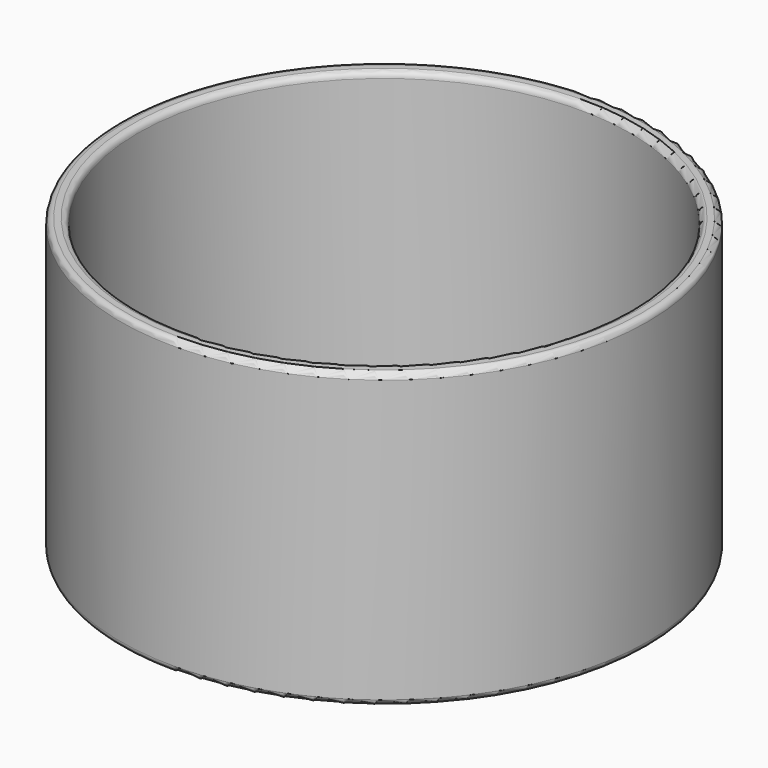
from build123d import *

# Parameters (mm, degrees)
F0_R     = 57.15
F1_DEPTH = 5.08
F2_R     = 1.27
F5_E1_W  = 63.5
F5_E1_H  = 3.81
F7_R     = 1.26999
F8_R     = 1.27


# Not quite as in the source:
# - a fillet or chamfer is up to 0.001 mm smaller than in the source, because OpenCascade refuses the exact size


with BuildPart() as f1:
    # F0 (on Top) → F1 (new body)
    with BuildSketch(Plane.XY):
        Circle(F0_R)
    extrude(amount=F1_DEPTH)

    # F2
    f2_edges = [f1.edges().sort_by_distance(p)[0] for p in [
        (-57.15, 0, 0),
    ]]
    fillet(f2_edges, radius=F2_R)

    # F5_E1 (on explicit) → F6 (revolve)
    with BuildSketch(Plane(origin=(57.15, 0, 0), x_dir=(0, 0, 1), z_dir=(0, -1, 0))):
        with Locations((31.75, 1.905)):
            Rectangle(F5_E1_W, F5_E1_H)
    revolve(axis=Axis((0, 0, 5.08), (0, 0, 1)))

    # F7 (radius 1.27 in the source; OpenCascade refuses exactly that, so slightly less here)
    f7_edges = [f1.edges().sort_by_distance(p)[0] for p in [
        (-57.15, 0, 0),
    ]]
    fillet(f7_edges, radius=F7_R)

    # F8
    f8_edges = [f1.edges().sort_by_distance(p)[0] for p in [
        (-57.15, 0, 63.5),
        (-53.34, 0, 63.5),
    ]]
    fillet(f8_edges, radius=F8_R)


solid = f1.part
